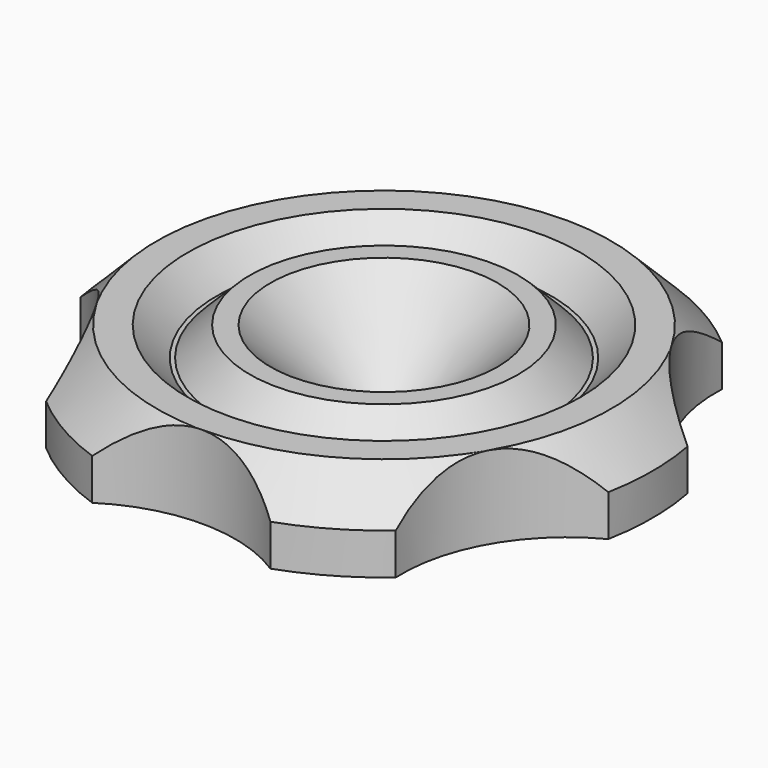
from build123d import *

# Parameters (mm, degrees)
F0_R            = 13
F1_DEPTH        = 4
F2_SIZE         = 2
F3_R            = 4.7
F4_DEPTH        = 2
F5_SIZE         = 0.5
F6_R            = 1.5
F7_DEPTH        = 25
F8_R            = 8
F9_DEPTH        = 25
F9_COPIES_COUNT = 6
F10_R           = 9.5
F10_R_2         = 6.5
F11_DEPTH       = 1.4
F12_SIZE        = 1.39999
F13_SIZE        = 4


# Not quite as in the source:
# - a fillet or chamfer is up to 0.001 mm smaller than in the source, because OpenCascade refuses the exact size
# - a pattern or mirror of a feature is missing from the dataset's text; its kind, count and spacing are read off the source's solid


with BuildPart() as f1:
    # F0 (on Top) → F1 (new body)
    with BuildSketch(Plane.XY):
        Circle(F0_R)
    extrude(amount=F1_DEPTH)

    # F2
    f2_edges = [f1.edges().sort_by_distance(p)[0] for p in [
        (-13, 0, 4),
    ]]
    chamfer(f2_edges, length=F2_SIZE)

    # F3 (on face) → F4 (join)
    with BuildSketch(Plane(origin=(0, 0, 0), x_dir=(1, 0, 0), z_dir=(0, 0, -1))):
        Circle(F3_R)
    extrude(amount=F4_DEPTH)

    # F5
    f5_edges = [f1.edges().sort_by_distance(p)[0] for p in [
        (-4.7, 0, -2),
    ]]
    chamfer(f5_edges, length=F5_SIZE)

    # F6 (on face) → F7 (cut)
    with BuildSketch(Plane(origin=(0, 0, -2), x_dir=(1, 0, 0), z_dir=(0, 0, -1))):
        Circle(F6_R)
    extrude(amount=-F7_DEPTH, mode=Mode.SUBTRACT)

    # F8 (on face) → F9 (cut)
    with BuildSketch(Plane(origin=(0, 0, 0), x_dir=(1, 0, 0), z_dir=(0, 0, -1))):
        with Locations((0, 19)):
            Circle(F8_R)
    f9 = extrude(amount=-F9_DEPTH, mode=Mode.SUBTRACT)

    # F9_copies: F9 ×6 about axis
    f9_copies_axis = Axis((0, 0, 0), (0, 0, 1))
    for i in range(1, F9_COPIES_COUNT):
        add(f9.rotate(f9_copies_axis, i * 360 / F9_COPIES_COUNT), mode=Mode.SUBTRACT)

    # F10 (on face) → F11 (cut)
    with BuildSketch(Plane.XY.offset(4)):
        Circle(F10_R)
        Circle(F10_R_2, mode=Mode.SUBTRACT)
    extrude(amount=-F11_DEPTH, mode=Mode.SUBTRACT)

    # F12 (size 1.4 in the source; OpenCascade refuses exactly that, so slightly less here)
    f12_edges = [f1.edges().sort_by_distance(p)[0] for p in [
        (-9.5, 0, 2.6),
        (-6.5, 0, 2.6),
    ]]
    chamfer(f12_edges, length=F12_SIZE)

    # F13
    f13_edges = [f1.edges().sort_by_distance(p)[0] for p in [
        (-1.5, 0, 4),
    ]]
    chamfer(f13_edges, length=F13_SIZE)


solid = f1.part
